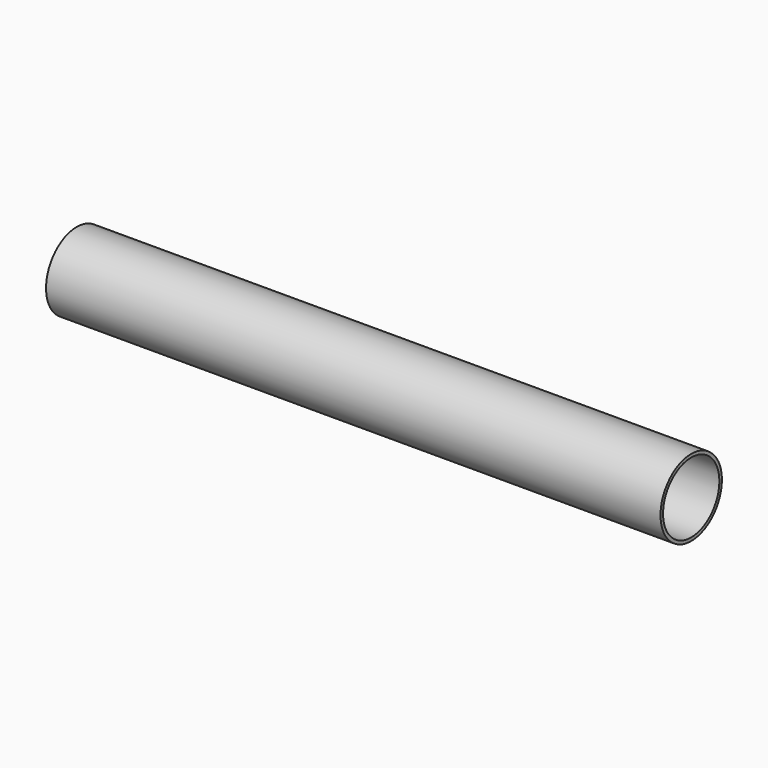
from build123d import *

# Parameters (mm, degrees)
F1_R     = 38.1
F1_R_2   = 34.925
F2_DEPTH = 609.6


# Not quite as in the source:
# - a variable given as a bare number and used for a length is read in inches; the dataset says mm whatever the document's units were


with BuildPart() as f2:
    # F1 (on Right) → F2 (new body)
    with BuildSketch(Plane.YZ):
        with Locations((13.9308627695, 20.094960928)):
            Circle(F1_R)
        with Locations((13.9308627695, 20.094960928)):
            Circle(F1_R_2, mode=Mode.SUBTRACT)
    extrude(amount=F2_DEPTH)


solid = f2.part
